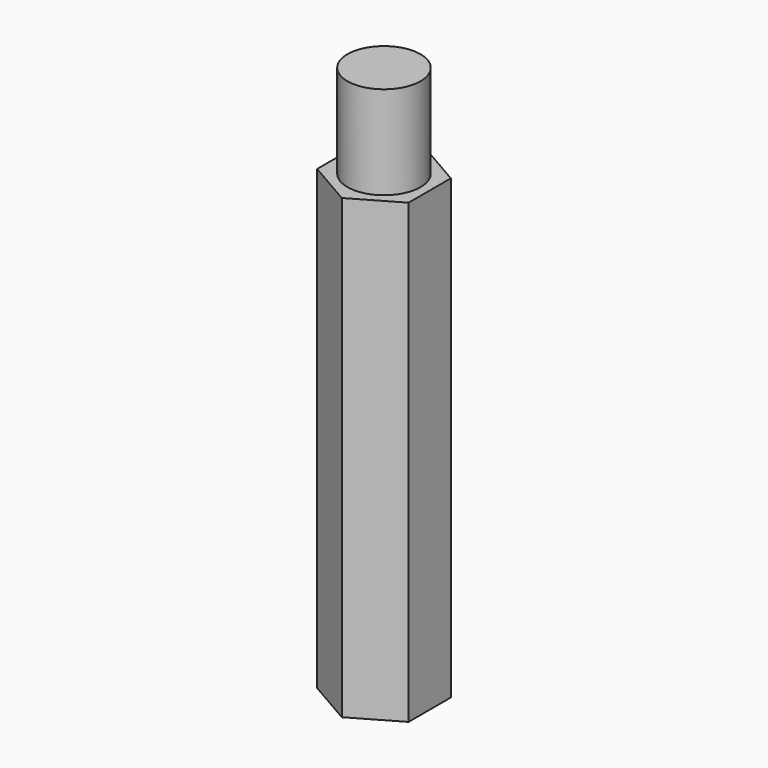
from build123d import *

# Parameters (mm, degrees)
F1_DEPTH = 25
F2_R     = 2
F3_DEPTH = 5.1
F4_R     = 2
F5_DEPTH = 10


with BuildPart() as f1:
    # F0 (on Top) → F1 (new body)
    with BuildSketch(Plane.XY):
        Polygon((2.5, 1.443375673), (0, 2.8867513459), (-2.5, 1.443375673), (-2.5, -1.443375673), (0, -2.8867513459), (2.5, -1.443375673), align=None)
    extrude(amount=F1_DEPTH)

    # F2 (on face) → F3 (join)
    with BuildSketch(Plane.XY.offset(25)):
        Circle(F2_R)
    extrude(amount=F3_DEPTH)

    # F4 (on face) → F5 (cut)
    with BuildSketch(Plane(origin=(0, 0, 0), x_dir=(1, 0, 0), z_dir=(0, 0, -1))):
        Circle(F4_R)
    extrude(amount=-F5_DEPTH, mode=Mode.SUBTRACT)


solid = f1.part
